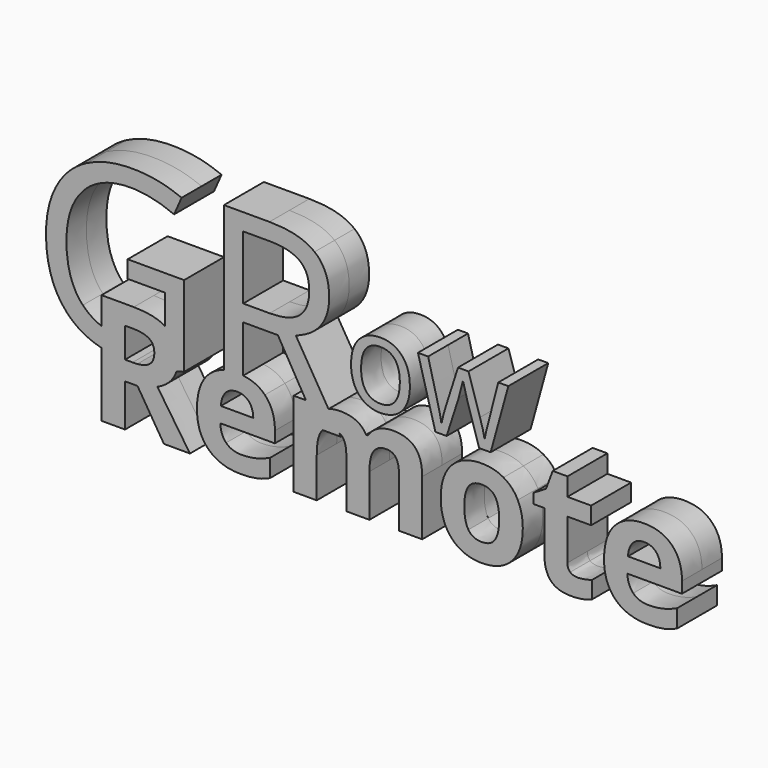
from build123d import *

# Parameters (mm, degrees)
F0_TEXT_SIZE = 15.2110267663
F1_DEPTH     = 3.175


# Not quite as in the source:
# - Text() gives the source's letters only with a copy of the font that has no kerning and outlines rounded to 1/6400 em; it was checked with that copy


with BuildPart() as f1:
    # F0 (on Front) → F1 (new body, symmetric)
    with BuildSketch(Plane.XZ):
        with BuildLine():
            Line((-18.0001128356, -0.1418109096), (-25.1771559294, -0.1418109096))
            Line((-25.1771559294, -0.1418109096), (-25.1771559294, -2.3369786298))
            Line((-25.1771559294, -2.3369786298), (-20.4587006823, -2.3369786298))
            Line((-20.4587006823, -2.3369786298), (-20.4587006823, -6.0761670225))
            add(Edge.make_bspline(
                [(-20.4587006823, -6.0761670225), (-20.2962684422, -6.1750486518), (-20.1506069671, -6.2856404547)],
                knots=[0.8941135468, 0.8941135468, 0.8941135468, 1, 1, 1], degree=2))
            add(Edge.make_bspline(
                [(-20.1506069671, -6.2856404547), (-18.7749685291, -7.330078149), (-18.7749685291, -9.4590057205)],
                knots=[0, 0, 0, 1, 1, 1], degree=2))
            add(Edge.make_bspline(
                [(-18.7749685291, -9.4590057205), (-18.7749685291, -10.1160833703), (-18.9660920729, -10.6963664585)],
                knots=[0, 0, 0, 0.5292109356, 0.5292109356, 0.5292109356], degree=2))
            add(Edge.make_bspline(
                [(-18.0001128356, -10.4105744346), (-18.4808256001, -10.5641906348), (-18.9660920729, -10.6963664585)],
                knots=[0, 0, 0, 0.2865529812, 0.2865529812, 0.2865529812], degree=2))
            Line((-18.0001128356, -10.4105744346), (-18.0001128356, -0.1418109096))
        make_face()
        with BuildLine():
            add(Edge.make_bspline(
                [(-18.9660920729, -10.6963664585), (-19.1361166667, -11.212589601), (-19.4573961081, -11.6680376579)],
                knots=[0.5292109356, 0.5292109356, 0.5292109356, 1, 1, 1], degree=2))
            add(Edge.make_bspline(
                [(-18.9660920729, -10.6963664585), (-20.17428721, -11.0254520154), (-21.410710262, -11.2216311397)],
                knots=[0.2865529812, 0.2865529812, 0.2865529812, 1, 1, 1], degree=2))
            add(Edge.make_bspline(
                [(-21.410710262, -11.2216311397), (-22.5596902038, -11.4039359571), (-23.9504027448, -11.4653744749)],
                knots=[0, 0, 0, 0.6629901576, 0.6629901576, 0.6629901576], degree=2))
            add(Edge.make_bspline(
                [(-24.5517256877, -11.4893433032), (-24.232147641, -11.4893433032), (-23.9504027448, -11.4653744749)],
                knots=[0, 0, 0, 0.2254946628, 0.2254946628, 0.2254946628], degree=2))
            Line((-24.5517256877, -11.4893433032), (-24.6992448802, -11.4893433032))
            add(Edge.make_bspline(
                [(-24.6992448802, -11.4893433032), (-25.0557168822, -11.4966047804), (-25.4267118386, -11.4966047804)],
                knots=[0.8374949138, 0.8374949138, 0.8374949138, 1, 1, 1], degree=2))
            add(Edge.make_bspline(
                [(-25.4267118386, -11.4966047804), (-27.0903738475, -11.4966047804), (-28.4984061784, -11.1527021089)],
                knots=[0, 0, 0, 0.3471460633, 0.3471460633, 0.3471460633], degree=2))
            Line((-28.4984061784, -11.1527021089), (-28.4984061784, -19.3180046044))
            Line((-28.4984061784, -19.3180046044), (-25.5129780788, -19.3180046044))
            Line((-25.5129780788, -19.3180046044), (-25.5129780788, -13.9171217783))
            Line((-25.5129780788, -13.9171217783), (-23.926295446, -13.9171217783))
            Line((-23.926295446, -13.9171217783), (-20.564993014, -19.3180046044))
            Line((-20.564993014, -19.3180046044), (-17.2529855764, -19.3180046044))
            add(Edge.make_bspline(
                [(-21.3937651077, -13.1838587363), (-18.2142379676, -17.9315828864), (-17.2529855764, -19.3180046044)],
                knots=[0, 0, 0, 1, 1, 1], degree=2))
            add(Edge.make_bspline(
                [(-19.4573961081, -11.6680376579), (-20.1398236871, -12.6354519234), (-21.3937651077, -13.1838587363)],
                knots=[0, 0, 0, 1, 1, 1], degree=2))
        make_face()
        with BuildLine():
            add(Edge.make_bspline(
                [(-18.9660920729, -10.6963664585), (-20.17428721, -11.0254520154), (-21.410710262, -11.2216311397)],
                knots=[0.2865529812, 0.2865529812, 0.2865529812, 1, 1, 1], degree=2))
            add(Edge.make_bspline(
                [(-18.7749685291, -9.4590057205), (-18.7749685291, -10.1160833703), (-18.9660920729, -10.6963664585)],
                knots=[0, 0, 0, 0.5292109356, 0.5292109356, 0.5292109356], degree=2))
            add(Edge.make_bspline(
                [(-20.1506069671, -6.2856404547), (-18.7749685291, -7.330078149), (-18.7749685291, -9.4590057205)],
                knots=[0, 0, 0, 1, 1, 1], degree=2))
            add(Edge.make_bspline(
                [(-20.4587006823, -6.0761670225), (-20.2962684422, -6.1750486518), (-20.1506069671, -6.2856404547)],
                knots=[0.8941135468, 0.8941135468, 0.8941135468, 1, 1, 1], degree=2))
            Line((-20.4587006823, -6.0761670225), (-20.4587006823, -8.8346750817))
            add(Edge.make_bspline(
                [(-21.8237577532, -9.1103678694), (-21.1359097556, -8.9991187861), (-20.4587006823, -8.8346750817)],
                knots=[0.6765177404, 0.6765177404, 0.6765177404, 1, 1, 1], degree=2))
            add(Edge.make_bspline(
                [(-21.788125063, -9.5360291493), (-21.788125063, -9.3082519111), (-21.8237577532, -9.1103678694)],
                knots=[0, 0, 0, 0.227480473, 0.227480473, 0.227480473], degree=2))
            add(Edge.make_bspline(
                [(-22.4613098306, -11.017959919), (-21.788125063, -10.5465765349), (-21.788125063, -9.5360291493)],
                knots=[0, 0, 0, 1, 1, 1], degree=2))
            add(Edge.make_bspline(
                [(-23.9504027448, -11.4653744749), (-22.9826950259, -11.3830488659), (-22.4613098306, -11.017959919)],
                knots=[0.2254946628, 0.2254946628, 0.2254946628, 1, 1, 1], degree=2))
            add(Edge.make_bspline(
                [(-21.410710262, -11.2216311397), (-22.5596902038, -11.4039359571), (-23.9504027448, -11.4653744749)],
                knots=[0, 0, 0, 0.6629901576, 0.6629901576, 0.6629901576], degree=2))
        make_face()
        with BuildLine():
            Line((-20.4587006823, -8.8346750817), (-20.4587006823, -6.0761670225))
            add(Edge.make_bspline(
                [(-24.3976788301, -5.2412027605), (-21.830291306, -5.2412027605), (-20.4587006823, -6.0761670225)],
                knots=[0, 0, 0, 0.8941135468, 0.8941135468, 0.8941135468], degree=2))
            Line((-24.3976788301, -5.2412027605), (-28.4984061784, -5.2412027605))
            Line((-28.4984061784, -5.2412027605), (-28.4984061784, -8.7168663055))
            add(Edge.make_bspline(
                [(-28.4984061784, -8.7168663055), (-27.1912605402, -9.2290174005), (-25.5129780788, -9.322270263)],
                knots=[0.4675941188, 0.4675941188, 0.4675941188, 0.9030591305, 0.9030591305, 0.9030591305], degree=2))
            Line((-25.5129780788, -9.322270263), (-25.5129780788, -7.6874668585))
            Line((-25.5129780788, -7.6874668585), (-24.6071825564, -7.6874668585))
            add(Edge.make_bspline(
                [(-22.4767145163, -8.1110957168), (-23.1653039696, -7.6874668585), (-24.6071825564, -7.6874668585)],
                knots=[0, 0, 0, 1, 1, 1], degree=2))
            add(Edge.make_bspline(
                [(-21.8237577532, -9.1103678694), (-21.9447657176, -8.4383572821), (-22.4767145163, -8.1110957168)],
                knots=[0.227480473, 0.227480473, 0.227480473, 1, 1, 1], degree=2))
            add(Edge.make_bspline(
                [(-21.8237577532, -9.1103678694), (-21.1359097556, -8.9991187861), (-20.4587006823, -8.8346750817)],
                knots=[0.6765177404, 0.6765177404, 0.6765177404, 1, 1, 1], degree=2))
        make_face()
        with BuildLine():
            add(Edge.make_bspline(
                [(-24.6992448802, -11.4893433032), (-25.0557168822, -11.4966047804), (-25.4267118386, -11.4966047804)],
                knots=[0.8374949138, 0.8374949138, 0.8374949138, 1, 1, 1], degree=2))
            Line((-24.6992448802, -11.4893433032), (-25.5129780788, -11.4893433032))
            Line((-25.5129780788, -11.4893433032), (-25.5129780788, -9.322270263))
            add(Edge.make_bspline(
                [(-28.4984061784, -8.7168663055), (-27.1912605402, -9.2290174005), (-25.5129780788, -9.322270263)],
                knots=[0.4675941188, 0.4675941188, 0.4675941188, 0.9030591305, 0.9030591305, 0.9030591305], degree=2))
            Line((-28.4984061784, -8.7168663055), (-28.4984061784, -11.1527021089))
            add(Edge.make_bspline(
                [(-25.4267118386, -11.4966047804), (-27.0903738475, -11.4966047804), (-28.4984061784, -11.1527021089)],
                knots=[0, 0, 0, 0.3471460633, 0.3471460633, 0.3471460633], degree=2))
        make_face()
        with BuildLine():
            Line((-28.4984061784, -11.1527021089), (-28.4984061784, -8.7168663055))
            add(Edge.make_bspline(
                [(-30.8776598934, -7.1339977743), (-29.901994518, -8.1669281164), (-28.4984061784, -8.7168663055)],
                knots=[0, 0, 0, 0.4675941188, 0.4675941188, 0.4675941188], degree=2))
            add(Edge.make_bspline(
                [(-32.9642245791, -0.6501655395), (-32.9642245791, -4.9249658368), (-30.8776598934, -7.1339977743)],
                knots=[0, 0, 0, 1, 1, 1], degree=2))
            add(Edge.make_bspline(
                [(-30.7967852932, 5.7204422549), (-32.9642245791, 3.4259143116), (-32.9642245791, -0.6501655395)],
                knots=[0, 0, 0, 1, 1, 1], degree=2))
            add(Edge.make_bspline(
                [(-24.7750936311, 8.0149701983), (-28.6293460073, 8.0149701983), (-30.7967852932, 5.7204422549)],
                knots=[0, 0, 0, 1, 1, 1], degree=2))
            add(Edge.make_bspline(
                [(-19.2709994105, 6.8041618979), (-22.1316495554, 8.0149701983), (-24.7750936311, 8.0149701983)],
                knots=[0, 0, 0, 1, 1, 1], degree=2))
            Line((-19.2709994105, 6.8041618979), (-18.3189898307, 8.9716011838))
            add(Edge.make_bspline(
                [(-24.6179658364, 10.2101379186), (-21.2350968444, 10.2101379186), (-18.3189898307, 8.9716011838)],
                knots=[0, 0, 0, 1, 1, 1], degree=2))
            add(Edge.make_bspline(
                [(-30.4340049436, 8.9045908007), (-27.9499993655, 10.2101379186), (-24.6179658364, 10.2101379186)],
                knots=[0, 0, 0, 1, 1, 1], degree=2))
            add(Edge.make_bspline(
                [(-34.2397325597, 5.1219702133), (-32.9180105218, 7.5990436829), (-30.4340049436, 8.9045908007)],
                knots=[0, 0, 0, 1, 1, 1], degree=2))
            add(Edge.make_bspline(
                [(-35.5614545976, -0.6501655395), (-35.5614545976, 2.6448967437), (-34.2397325597, 5.1219702133)],
                knots=[0, 0, 0, 1, 1, 1], degree=2))
            add(Edge.make_bspline(
                [(-32.8902820875, -8.6428867441), (-35.5614545976, -5.7891687078), (-35.5614545976, -0.6501655395)],
                knots=[0, 0, 0, 1, 1, 1], degree=2))
            add(Edge.make_bspline(
                [(-28.4984061784, -11.1527021089), (-31.1463965987, -10.5059477982), (-32.8902820875, -8.6428867441)],
                knots=[0.3471460633, 0.3471460633, 0.3471460633, 1, 1, 1], degree=2))
        make_face()
        with BuildLine():
            Line((-10.481085718, -8.395441166), (-10.481085718, -2.4247853386))
            Line((-10.481085718, -2.4247853386), (-6.0722646546, -2.4247853386))
            Line((-6.0722646546, -2.4247853386), (-2.5048762891, -8.553210198))
            Line((-2.5048762891, -8.553210198), (-1.8205713859, -8.553210198))
            Line((-1.8205713859, -8.553210198), (-1.4262114305, -9.9303891046))
            Line((-1.4262114305, -9.9303891046), (-1.2629217615, -9.9303891046))
            add(Edge.make_bspline(
                [(-1.2629217615, -9.9303891046), (-0.8285096232, -9.1878832512), (-0.0105208096, -8.7704162672)],
                knots=[0, 0, 0, 1, 1, 1], degree=2))
            add(Edge.make_bspline(
                [(-0.0105208096, -8.7704162672), (0.1730350404, -8.6767371046), (0.3687694022, -8.60407945)],
                knots=[0, 0, 0, 0.2243989732, 0.2243989732, 0.2243989732], degree=2))
            Line((0.3687694022, -8.60407945), (-3.7939116313, -1.7177102624))
            add(Edge.make_bspline(
                [(0.4531602317, 3.943511753), (0.4531602317, -0.2434818355), (-3.7939116313, -1.7177102624)],
                knots=[0, 0, 0, 1, 1, 1], degree=2))
            add(Edge.make_bspline(
                [(-1.4023341676, 8.4216539023), (0.4531602317, 6.9335612582), (0.4531602317, 3.943511753)],
                knots=[0, 0, 0, 1, 1, 1], degree=2))
            add(Edge.make_bspline(
                [(-7.1444307832, 9.9097465463), (-3.257828567, 9.9097465463), (-1.4023341676, 8.4216539023)],
                knots=[0, 0, 0, 1, 1, 1], degree=2))
            Line((-7.1444307832, 9.9097465463), (-12.935052159, 9.9097465463))
            Line((-12.935052159, 9.9097465463), (-12.935052159, -8.5654224954))
            add(Edge.make_bspline(
                [(-12.935052159, -8.5654224954), (-12.1784125316, -8.3529492832), (-11.2728865659, -8.3529492832)],
                knots=[0.6207580539, 0.6207580539, 0.6207580539, 1, 1, 1], degree=2))
            add(Edge.make_bspline(
                [(-11.2728865659, -8.3529492832), (-10.8604783227, -8.3529492832), (-10.481085718, -8.395441166)],
                knots=[0, 0, 0, 0.1808892585, 0.1808892585, 0.1808892585], degree=2))
        make_face()
        with BuildLine():
            Line((-7.1120809431, -0.3174243272), (-10.481085718, -0.3174243272))
            Line((-10.481085718, -0.3174243272), (-10.481085718, 7.7561714776))
            Line((-10.481085718, 7.7561714776), (-7.2876943608, 7.7561714776))
            add(Edge.make_bspline(
                [(-3.3225282471, 6.8318903323), (-4.5564435762, 7.7561714776), (-7.2876943608, 7.7561714776)],
                knots=[0, 0, 0, 1, 1, 1], degree=2))
            add(Edge.make_bspline(
                [(-2.0886129181, 3.8141123926), (-2.0886129181, 5.9076091869), (-3.3225282471, 6.8318903323)],
                knots=[0, 0, 0, 1, 1, 1], degree=2))
            add(Edge.make_bspline(
                [(-3.3017319214, 0.7154598528), (-2.0886129181, 1.7483440327), (-2.0886129181, 3.8141123926)],
                knots=[0, 0, 0, 1, 1, 1], degree=2))
            add(Edge.make_bspline(
                [(-7.1120809431, -0.3174243272), (-4.5148509247, -0.3174243272), (-3.3017319214, 0.7154598528)],
                knots=[0, 0, 0, 1, 1, 1], degree=2))
        make_face(mode=Mode.SUBTRACT)
        with BuildLine():
            add(Edge.make_bspline(
                [(-10.481085718, -8.395441166), (-8.7631033438, -8.5878547893), (-7.7221064991, -9.6515642925)],
                knots=[0.1808892585, 0.1808892585, 0.1808892585, 1, 1, 1], degree=2))
            Line((-10.481085718, -8.395441166), (-10.481085718, -10.565547728))
            add(Edge.make_bspline(
                [(-9.7724701732, -11.0333646048), (-10.0700720225, -10.7123558685), (-10.481085718, -10.565547728)],
                knots=[0, 0, 0, 0.5426662147, 0.5426662147, 0.5426662147], degree=2))
            add(Edge.make_bspline(
                [(-9.2024968002, -12.7124753522), (-9.2240633603, -11.6249045378), (-9.7724701732, -11.0333646048)],
                knots=[0, 0, 0, 1, 1, 1], degree=2))
            Line((-9.2024968002, -12.7124753522), (-13.3247907086, -12.7124753522))
            add(Edge.make_bspline(
                [(-12.8550402063, -11.2054562196), (-13.2583603391, -11.7744785346), (-13.3247907086, -12.7124753522)],
                knots=[0.1375303519, 0.1375303519, 0.1375303519, 1, 1, 1], degree=2))
            Line((-12.8550402063, -11.2054562196), (-12.935052159, -11.2054562196))
            Line((-12.935052159, -11.2054562196), (-12.935052159, -8.5654224954))
            add(Edge.make_bspline(
                [(-15.0131442675, -9.8302586472), (-14.1735495019, -8.9132069614), (-12.935052159, -8.5654224954)],
                knots=[0, 0, 0, 0.6207580539, 0.6207580539, 0.6207580539], degree=2))
            add(Edge.make_bspline(
                [(-16.3656756769, -14.01263083), (-16.3656756769, -11.3075680112), (-15.0131442675, -9.8302586472)],
                knots=[0, 0, 0, 1, 1, 1], degree=2))
            add(Edge.make_bspline(
                [(-14.90223053, -18.0763869325), (-16.3656756769, -16.64067022), (-16.3656756769, -14.01263083)],
                knots=[0, 0, 0, 1, 1, 1], degree=2))
            add(Edge.make_bspline(
                [(-10.8415553647, -19.512103645), (-13.4387853832, -19.512103645), (-14.90223053, -18.0763869325)],
                knots=[0, 0, 0, 1, 1, 1], degree=2))
            add(Edge.make_bspline(
                [(-8.7033849817, -19.3241664787), (-9.5783711327, -19.512103645), (-10.8415553647, -19.512103645)],
                knots=[0, 0, 0, 1, 1, 1], degree=2))
            add(Edge.make_bspline(
                [(-7.058164543, -18.7511121686), (-7.8283988308, -19.1362293125), (-8.7033849817, -19.3241664787)],
                knots=[0, 0, 0, 1, 1, 1], degree=2))
            Line((-7.058164543, -18.7511121686), (-7.058164543, -16.477380551))
            add(Edge.make_bspline(
                [(-8.8666746508, -17.1228368842), (-8.0009313113, -16.9210355008), (-7.058164543, -16.477380551)],
                knots=[0, 0, 0, 1, 1, 1], degree=2))
            add(Edge.make_bspline(
                [(-10.70599413, -17.3246382676), (-9.7324179903, -17.3246382676), (-8.8666746508, -17.1228368842)],
                knots=[0, 0, 0, 1, 1, 1], degree=2))
            add(Edge.make_bspline(
                [(-12.6500654725, -16.6221845971), (-11.9568546134, -17.3246382676), (-10.70599413, -17.3246382676)],
                knots=[0, 0, 0, 1, 1, 1], degree=2))
            add(Edge.make_bspline(
                [(-13.3925713259, -14.6688704432), (-13.3432763315, -15.9197309266), (-12.6500654725, -16.6221845971)],
                knots=[0, 0, 0, 1, 1, 1], degree=2))
            Line((-13.3925713259, -14.6688704432), (-6.4512199242, -14.6688704432))
            Line((-6.4512199242, -14.6688704432), (-6.4512199242, -13.2423965422))
            add(Edge.make_bspline(
                [(-7.7221064991, -9.6515642925), (-6.4512199242, -10.9501793017), (-6.4512199242, -13.2423965422)],
                knots=[0, 0, 0, 1, 1, 1], degree=2))
        make_face()
        with BuildLine():
            Line((-10.481085718, -10.565547728), (-10.481085718, -8.395441166))
            add(Edge.make_bspline(
                [(-11.2728865659, -8.3529492832), (-10.8604783227, -8.3529492832), (-10.481085718, -8.395441166)],
                knots=[0, 0, 0, 0.1808892585, 0.1808892585, 0.1808892585], degree=2))
            add(Edge.make_bspline(
                [(-12.935052159, -8.5654224954), (-12.1784125316, -8.3529492832), (-11.2728865659, -8.3529492832)],
                knots=[0.6207580539, 0.6207580539, 0.6207580539, 1, 1, 1], degree=2))
            Line((-12.935052159, -8.5654224954), (-12.935052159, -11.2054562196))
            Line((-12.935052159, -11.2054562196), (-12.8550402063, -11.2054562196))
            add(Edge.make_bspline(
                [(-12.7178460898, -11.0333646048), (-12.7907263375, -11.1147192999), (-12.8550402063, -11.2054562196)],
                knots=[0, 0, 0, 0.1375303519, 0.1375303519, 0.1375303519], degree=2))
            add(Edge.make_bspline(
                [(-11.254400943, -10.4418246717), (-12.1879248998, -10.4418246717), (-12.7178460898, -11.0333646048)],
                knots=[0, 0, 0, 1, 1, 1], degree=2))
            add(Edge.make_bspline(
                [(-10.481085718, -10.565547728), (-10.8274688981, -10.4418246717), (-11.254400943, -10.4418246717)],
                knots=[0.5426662147, 0.5426662147, 0.5426662147, 1, 1, 1], degree=2))
        make_face()
        with BuildLine():
            Line((-1.8205713859, -8.553210198), (-2.5048762891, -8.553210198))
            Line((-2.5048762891, -8.553210198), (-0.9609899207, -11.2054562196))
            Line((-0.9609899207, -11.2054562196), (-0.3638205123, -11.2054562196))
            add(Edge.make_bspline(
                [(1.0200526675, -10.7006233924), (0.1399767062, -10.7006233924), (-0.3638205123, -11.2054562196)],
                knots=[0, 0, 0, 0.780470036, 0.780470036, 0.780470036], degree=2))
            add(Edge.make_bspline(
                [(1.7156849005, -10.832296628), (1.4185525294, -10.7006233924), (1.0200526675, -10.7006233924)],
                knots=[0.5244716299, 0.5244716299, 0.5244716299, 1, 1, 1], degree=2))
            Line((1.7156849005, -10.832296628), (0.3687694022, -8.60407945))
            add(Edge.make_bspline(
                [(-0.0105208096, -8.7704162672), (0.1730350404, -8.6767371046), (0.3687694022, -8.60407945)],
                knots=[0, 0, 0, 0.2243989732, 0.2243989732, 0.2243989732], degree=2))
            add(Edge.make_bspline(
                [(-1.2629217615, -9.9303891046), (-0.8285096232, -9.1878832512), (-0.0105208096, -8.7704162672)],
                knots=[0, 0, 0, 1, 1, 1], degree=2))
            Line((-1.2629217615, -9.9303891046), (-1.4262114305, -9.9303891046))
            Line((-1.4262114305, -9.9303891046), (-1.8205713859, -8.553210198))
        make_face()
        with BuildLine():
            Line((-0.9609899207, -11.2054562196), (-2.5048762891, -8.553210198))
            Line((-2.5048762891, -8.553210198), (-4.063493632, -8.553210198))
            Line((-4.063493632, -8.553210198), (-4.063493632, -19.3180046044))
            Line((-4.063493632, -19.3180046044), (-1.1273605269, -19.3180046044))
            Line((-1.1273605269, -19.3180046044), (-1.1273605269, -14.2529439278))
            add(Edge.make_bspline(
                [(-0.6174654284, -11.5293954861), (-1.1273605269, -12.3581675798), (-1.1273605269, -14.2529439278)],
                knots=[0, 0, 0, 1, 1, 1], degree=2))
            add(Edge.make_bspline(
                [(-0.3638205123, -11.2054562196), (-0.5055281757, -11.3474551783), (-0.6174654284, -11.5293954861)],
                knots=[0.780470036, 0.780470036, 0.780470036, 1, 1, 1], degree=2))
            Line((-0.3638205123, -11.2054562196), (-0.9609899207, -11.2054562196))
        make_face()
        with BuildLine():
            add(Edge.make_bspline(
                [(1.0200526675, -10.7006233924), (0.1399767062, -10.7006233924), (-0.3638205123, -11.2054562196)],
                knots=[0, 0, 0, 0.780470036, 0.780470036, 0.780470036], degree=2))
            Line((-0.3638205123, -11.2054562196), (1.9412528757, -11.2054562196))
            Line((1.9412528757, -11.2054562196), (1.7156849005, -10.832296628))
            add(Edge.make_bspline(
                [(1.7156849005, -10.832296628), (1.4185525294, -10.7006233924), (1.0200526675, -10.7006233924)],
                knots=[0.5244716299, 0.5244716299, 0.5244716299, 1, 1, 1], degree=2))
        make_face()
        with BuildLine():
            Line((0.3687694022, -8.60407945), (1.7156849005, -10.832296628))
            add(Edge.make_bspline(
                [(2.2478061223, -11.282920514), (2.0433993099, -10.9775221936), (1.7156849005, -10.832296628)],
                knots=[0, 0, 0, 0.5244716299, 0.5244716299, 0.5244716299], degree=2))
            add(Edge.make_bspline(
                [(2.6375446719, -13.0298118788), (2.6375446719, -11.8652176356), (2.2478061223, -11.282920514)],
                knots=[0, 0, 0, 1, 1, 1], degree=2))
            Line((2.6375446719, -13.0298118788), (2.6375446719, -19.3180046044))
            Line((2.6375446719, -19.3180046044), (5.573677777, -19.3180046044))
            Line((5.573677777, -19.3180046044), (5.573677777, -13.9171217783))
            add(Edge.make_bspline(
                [(6.1082203728, -11.4708576803), (5.573677777, -12.2410919681), (5.573677777, -13.9171217783)],
                knots=[0, 0, 0, 1, 1, 1], degree=2))
            add(Edge.make_bspline(
                [(7.7210909714, -10.7006233924), (6.6427629685, -10.7006233924), (6.1082203728, -11.4708576803)],
                knots=[0, 0, 0, 1, 1, 1], degree=2))
            add(Edge.make_bspline(
                [(8.9488444262, -11.282920514), (8.5591058766, -10.7006233924), (7.7210909714, -10.7006233924)],
                knots=[0, 0, 0, 1, 1, 1], degree=2))
            add(Edge.make_bspline(
                [(9.3385829758, -13.0298118788), (9.3385829758, -11.8652176356), (8.9488444262, -11.282920514)],
                knots=[0, 0, 0, 1, 1, 1], degree=2))
            Line((9.3385829758, -13.0298118788), (9.3385829758, -19.3180046044))
            Line((9.3385829758, -19.3180046044), (12.2839588924, -19.3180046044))
            Line((12.2839588924, -19.3180046044), (12.2839588924, -12.2996297739))
            add(Edge.make_bspline(
                [(11.3458135299, -9.2910946458), (12.2839588924, -10.2292400083), (12.2839588924, -12.2996297739)],
                knots=[0, 0, 0, 1, 1, 1], degree=2))
            add(Edge.make_bspline(
                [(8.5775914995, -8.3529492832), (10.4076681673, -8.3529492832), (11.3458135299, -9.2910946458)],
                knots=[0, 0, 0, 1, 1, 1], degree=2))
            add(Edge.make_bspline(
                [(6.6766532772, -8.7657948615), (7.5177491195, -8.3529492832), (8.5775914995, -8.3529492832)],
                knots=[0, 0, 0, 1, 1, 1], degree=2))
            add(Edge.make_bspline(
                [(5.4011452966, -9.9303891046), (5.8355574349, -9.1786404397), (6.6766532772, -8.7657948615)],
                knots=[0, 0, 0, 1, 1, 1], degree=2))
            Line((5.4011452966, -9.9303891046), (5.1423465759, -9.9303891046))
            add(Edge.make_bspline(
                [(1.8673103841, -8.3529492832), (4.2827651107, -8.3529492832), (5.1423465759, -9.9303891046)],
                knots=[0, 0, 0, 1, 1, 1], degree=2))
            add(Edge.make_bspline(
                [(0.3687694022, -8.60407945), (1.045295546, -8.3529492832), (1.8673103841, -8.3529492832)],
                knots=[0.2243989732, 0.2243989732, 0.2243989732, 1, 1, 1], degree=2))
        make_face()
        with BuildLine():
            add(Edge.make_bspline(
                [(25.0790908815, -13.9171217783), (25.0790908815, -16.5451611683), (23.6926691634, -18.0286324066)],
                knots=[0, 0, 0, 1, 1, 1], degree=2))
            add(Edge.make_bspline(
                [(24.4444178283, -10.9609625817), (25.0790908815, -12.2226063452), (25.0790908815, -13.9171217783)],
                knots=[0, 0, 0, 1, 1, 1], degree=2))
            add(Edge.make_bspline(
                [(22.6251244405, -9.0261340508), (23.8097447752, -9.6993188183), (24.4444178283, -10.9609625817)],
                knots=[0, 0, 0, 1, 1, 1], degree=2))
            add(Edge.make_bspline(
                [(19.8907927188, -8.3529492832), (21.4405041059, -8.3529492832), (22.6251244405, -9.0261340508)],
                knots=[0, 0, 0, 1, 1, 1], degree=2))
            add(Edge.make_bspline(
                [(16.0195951883, -9.81639443), (17.3952336263, -8.3529492832), (19.8907927188, -8.3529492832)],
                knots=[0, 0, 0, 1, 1, 1], degree=2))
            add(Edge.make_bspline(
                [(14.6439567503, -13.9171217783), (14.6439567503, -11.2798395769), (16.0195951883, -9.81639443)],
                knots=[0, 0, 0, 1, 1, 1], degree=2))
            add(Edge.make_bspline(
                [(15.2786298034, -16.8825237864), (14.6439567503, -15.6116372115), (14.6439567503, -13.9171217783)],
                knots=[0, 0, 0, 1, 1, 1], degree=2))
            add(Edge.make_bspline(
                [(17.0979231912, -18.8327570031), (15.9133028566, -18.1534103613), (15.2786298034, -16.8825237864)],
                knots=[0, 0, 0, 1, 1, 1], degree=2))
            add(Edge.make_bspline(
                [(19.8322549129, -19.512103645), (18.2825435259, -19.512103645), (17.0979231912, -18.8327570031)],
                knots=[0, 0, 0, 1, 1, 1], degree=2))
            add(Edge.make_bspline(
                [(23.6926691634, -18.0286324066), (22.3062474454, -19.512103645), (19.8322549129, -19.512103645)],
                knots=[0, 0, 0, 1, 1, 1], degree=2))
        make_face()
        with BuildLine():
            add(Edge.make_bspline(
                [(17.6355467241, -13.9171217783), (17.6355467241, -15.5161281598), (18.1608465084, -16.3341169735)],
                knots=[0, 0, 0, 1, 1, 1], degree=2))
            add(Edge.make_bspline(
                [(18.1562251027, -11.5139908004), (17.6355467241, -12.3088725854), (17.6355467241, -13.9171217783)],
                knots=[0, 0, 0, 1, 1, 1], degree=2))
            add(Edge.make_bspline(
                [(19.8507405358, -10.7191090154), (18.6769034812, -10.7191090154), (18.1562251027, -11.5139908004)],
                knots=[0, 0, 0, 1, 1, 1], degree=2))
            add(Edge.make_bspline(
                [(21.556039249, -11.5186122061), (21.0369013391, -10.7191090154), (19.8507405358, -10.7191090154)],
                knots=[0, 0, 0, 1, 1, 1], degree=2))
            add(Edge.make_bspline(
                [(22.075177159, -13.9171217783), (22.075177159, -12.3181153968), (21.556039249, -11.5186122061)],
                knots=[0, 0, 0, 1, 1, 1], degree=2))
            add(Edge.make_bspline(
                [(21.5606606548, -16.3387383792), (22.075177159, -15.5253709713), (22.075177159, -13.9171217783)],
                knots=[0, 0, 0, 1, 1, 1], degree=2))
            add(Edge.make_bspline(
                [(19.8692261587, -17.1521057871), (21.0461441505, -17.1521057871), (21.5606606548, -16.3387383792)],
                knots=[0, 0, 0, 1, 1, 1], degree=2))
            add(Edge.make_bspline(
                [(18.1608465084, -16.3341169735), (18.6861462927, -17.1521057871), (19.8692261587, -17.1521057871)],
                knots=[0, 0, 0, 1, 1, 1], degree=2))
        make_face(mode=Mode.SUBTRACT)
        with BuildLine():
            add(Edge.make_bspline(
                [(32.0420088432, -17.17059141), (32.812243131, -17.17059141), (33.890571134, -16.8347692605)],
                knots=[0, 0, 0, 1, 1, 1], degree=2))
            add(Edge.make_bspline(
                [(31.1115658236, -16.8717405064), (31.4627926588, -17.17059141), (32.0420088432, -17.17059141)],
                knots=[0, 0, 0, 1, 1, 1], degree=2))
            add(Edge.make_bspline(
                [(30.7603389883, -15.947459361), (30.7603389883, -16.5728896027), (31.1115658236, -16.8717405064)],
                knots=[0, 0, 0, 1, 1, 1], degree=2))
            Line((30.7603389883, -15.947459361), (30.7603389883, -10.7591611983))
            Line((30.7603389883, -10.7591611983), (33.7734955222, -10.7591611983))
            Line((33.7734955222, -10.7591611983), (33.7734955222, -8.553210198))
            Line((33.7734955222, -8.553210198), (30.7603389883, -8.553210198))
            Line((30.7603389883, -8.553210198), (30.7603389883, -6.2609929575))
            Line((30.7603389883, -6.2609929575), (28.8840482632, -6.2609929575))
            Line((28.8840482632, -6.2609929575), (28.0367905466, -8.5347245751))
            Line((28.0367905466, -8.5347245751), (26.4192985422, -9.5175435264))
            Line((26.4192985422, -9.5175435264), (26.4192985422, -10.7591611983))
            Line((26.4192985422, -10.7591611983), (27.8242058832, -10.7591611983))
            Line((27.8242058832, -10.7591611983), (27.8242058832, -15.947459361))
            add(Edge.make_bspline(
                [(28.6283304797, -18.6201723397), (27.8242058832, -17.7282410344), (27.8242058832, -15.947459361)],
                knots=[0, 0, 0, 1, 1, 1], degree=2))
            add(Edge.make_bspline(
                [(31.1947511267, -19.512103645), (29.4324550762, -19.512103645), (28.6283304797, -18.6201723397)],
                knots=[0, 0, 0, 1, 1, 1], degree=2))
            add(Edge.make_bspline(
                [(33.890571134, -19.0191537008), (32.7937575081, -19.512103645), (31.1947511267, -19.512103645)],
                knots=[0, 0, 0, 1, 1, 1], degree=2))
            Line((33.890571134, -19.0191537008), (33.890571134, -16.8347692605))
        make_face()
        with BuildLine():
            add(Edge.make_bspline(
                [(40.9366743988, -19.512103645), (38.3394443804, -19.512103645), (36.8759992335, -18.0763869325)],
                knots=[0, 0, 0, 1, 1, 1], degree=2))
            add(Edge.make_bspline(
                [(43.0748447818, -19.3241664787), (42.1998586308, -19.512103645), (40.9366743988, -19.512103645)],
                knots=[0, 0, 0, 1, 1, 1], degree=2))
            add(Edge.make_bspline(
                [(44.7200652205, -18.7511121686), (43.9498309327, -19.1362293125), (43.0748447818, -19.3241664787)],
                knots=[0, 0, 0, 1, 1, 1], degree=2))
            Line((44.7200652205, -18.7511121686), (44.7200652205, -16.477380551))
            add(Edge.make_bspline(
                [(42.9115551128, -17.1228368842), (43.7772984523, -16.9210355008), (44.7200652205, -16.477380551)],
                knots=[0, 0, 0, 1, 1, 1], degree=2))
            add(Edge.make_bspline(
                [(41.0722356335, -17.3246382676), (42.0458117733, -17.3246382676), (42.9115551128, -17.1228368842)],
                knots=[0, 0, 0, 1, 1, 1], degree=2))
            add(Edge.make_bspline(
                [(39.1281642911, -16.6221845971), (39.8213751501, -17.3246382676), (41.0722356335, -17.3246382676)],
                knots=[0, 0, 0, 1, 1, 1], degree=2))
            add(Edge.make_bspline(
                [(38.3856584376, -14.6688704432), (38.434953432, -15.9197309266), (39.1281642911, -16.6221845971)],
                knots=[0, 0, 0, 1, 1, 1], degree=2))
            Line((38.3856584376, -14.6688704432), (45.3270098393, -14.6688704432))
            Line((45.3270098393, -14.6688704432), (45.3270098393, -13.2423965422))
            add(Edge.make_bspline(
                [(44.0561232645, -9.6515642925), (45.3270098393, -10.9501793017), (45.3270098393, -13.2423965422)],
                knots=[0, 0, 0, 1, 1, 1], degree=2))
            add(Edge.make_bspline(
                [(40.5053431977, -8.3529492832), (42.7852366896, -8.3529492832), (44.0561232645, -9.6515642925)],
                knots=[0, 0, 0, 1, 1, 1], degree=2))
            add(Edge.make_bspline(
                [(36.7650854961, -9.8302586472), (38.1176169055, -8.3529492832), (40.5053431977, -8.3529492832)],
                knots=[0, 0, 0, 1, 1, 1], degree=2))
            add(Edge.make_bspline(
                [(35.4125540867, -14.01263083), (35.4125540867, -11.3075680112), (36.7650854961, -9.8302586472)],
                knots=[0, 0, 0, 1, 1, 1], degree=2))
            add(Edge.make_bspline(
                [(36.8759992335, -18.0763869325), (35.4125540867, -16.64067022), (35.4125540867, -14.01263083)],
                knots=[0, 0, 0, 1, 1, 1], degree=2))
        make_face()
        with BuildLine():
            add(Edge.make_bspline(
                [(40.5238288206, -10.4418246717), (39.5903048637, -10.4418246717), (39.0603836737, -11.0333646048)],
                knots=[0, 0, 0, 1, 1, 1], degree=2))
            add(Edge.make_bspline(
                [(42.0057595903, -11.0333646048), (41.4573527774, -10.4418246717), (40.5238288206, -10.4418246717)],
                knots=[0, 0, 0, 1, 1, 1], degree=2))
            add(Edge.make_bspline(
                [(42.5757329633, -12.7124753522), (42.5541664032, -11.6249045378), (42.0057595903, -11.0333646048)],
                knots=[0, 0, 0, 1, 1, 1], degree=2))
            Line((42.5757329633, -12.7124753522), (38.4534390549, -12.7124753522))
            add(Edge.make_bspline(
                [(39.0603836737, -11.0333646048), (38.5304624837, -11.6249045378), (38.4534390549, -12.7124753522)],
                knots=[0, 0, 0, 1, 1, 1], degree=2))
        make_face(mode=Mode.SUBTRACT)
        with Locations((2.3830591235, -6.7435554229)):
            Text('ow', F0_TEXT_SIZE, font='Open Sans', text_align=(TextAlign.LEFT, TextAlign.BOTTOM))
    extrude(amount=F1_DEPTH, both=True)


solid = f1.part
